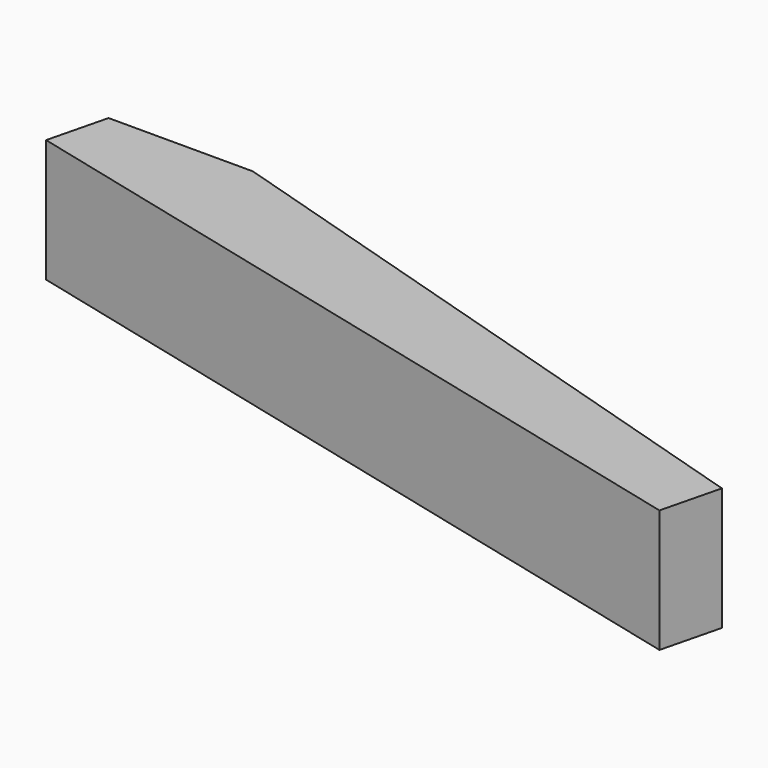
from build123d import *

# Parameters (mm, degrees)
F2_DEPTH = 25.4
F3_DEPTH = 12.7


# Not quite as in the source:
# - a length typed as a fraction of an inch, garbled in the dataset ("3 / 203.2 mm" for 3/8 in), is restored


with BuildPart() as f2:
    # F1 (on face) → F2 (new body)
    with BuildSketch(Plane.XY):
        Polygon((-29.84200418, 14.5122259855), (128.3614784479, -24.7320532799), (0, 14.5122259855), align=None)
    extrude(amount=F2_DEPTH)

    # F3 (add): a face of the model
    f3_faces = [f2.faces().sort_by_distance(p)[0] for p in [
        (49.259737134, -5.1099136472, 12.7),
    ]]
    extrude(f3_faces, amount=F3_DEPTH)


solid = f2.part
